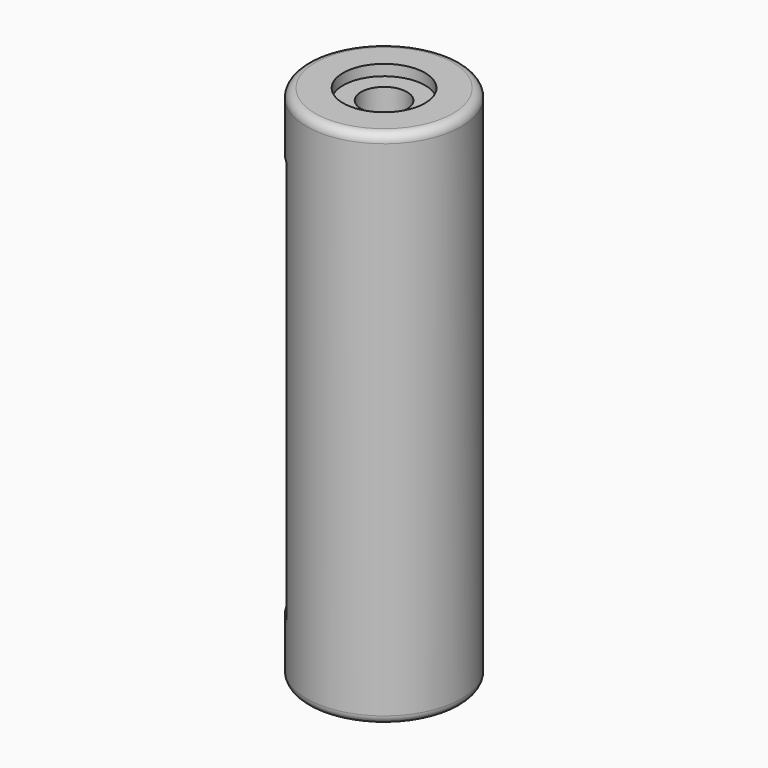
from build123d import *

# Parameters (mm, degrees)
F0_R          = 7.1
F0_R_2        = 2.1
F1_DEPTH      = 47.7
F3_DEPTH      = 3.2
F4_R          = 3.75
F5_DEPTH      = 1
F6_W          = 8
F6_H          = 35.7
F7_DEPTH      = 25
F9_START      = -2.5
F8_R          = 5.1
F9_DEPTH      = 37.5
F10_T1_DEPTH  = 35.7
F10_T8_ANGLE  = 100.8666218277
F10_T14_ANGLE = 100.8666218277
F10_T23_DEPTH = 40.4388611997
F10_T27_ANGLE = 100.8666218277
F10_T34_ANGLE = 100.8666218277
F10_T38_DEPTH = 40.4388611997
F10_T45_DEPTH = 40.4388611997
F10_T49_ANGLE = 100.8666218277
F10_T56_DEPTH = 40.4388611997
F10_T60_ANGLE = 100.8666218277


# Not quite as in the source:
# - a fillet or chamfer that OpenCascade refuses, or shapes differently, is made with other operations: its cross-section is extruded or revolved along the edge and cut away or added


with BuildPart() as f1:
    # F0 (on Top) → F1 (new body)
    with BuildSketch(Plane.XY):
        Circle(F0_R)
        Circle(F0_R_2, mode=Mode.SUBTRACT)
    extrude(amount=F1_DEPTH)

    # F2 (on face) → F3 (cut)
    with BuildSketch(Plane(origin=(0, 0, 0), x_dir=(1, 0, 0), z_dir=(0, 0, -1))):
        Polygon((2.6088002978, -3.8114950268), (4.6052516685, 0.3535398179), (1.9964513707, 4.1650348447), (-2.6088002978, 3.8114950268), (-4.6052516685, -0.3535398179), (-1.9964513707, -4.1650348447), align=None)
    extrude(amount=-F3_DEPTH, mode=Mode.SUBTRACT)

    # F4 (on face) → F5 (cut)
    with BuildSketch(Plane.XY.offset(47.7)):
        Circle(F4_R)
    extrude(amount=-F5_DEPTH, mode=Mode.SUBTRACT)

    # F6 (on Right) → F7 (cut)
    with BuildSketch(Plane.YZ):
        with Locations((0, 23.85)):
            Rectangle(F6_W, F6_H)
    extrude(amount=-F7_DEPTH, mode=Mode.SUBTRACT)

    # F8 (on face) → F9 (cut)
    with BuildSketch(Plane(origin=(0, 0, 3.2), x_dir=(1, 0, 0), z_dir=(0, 0, -1)).offset(F9_START)):
        Circle(F8_R)
    extrude(amount=-F9_DEPTH, mode=Mode.SUBTRACT)

    # F10: fillet of radius 0.8 on 6 edges, made by hand

    # F10_s2 → F10_t1 (cut)
    with BuildSketch(Plane.XY.offset(6)):
        with BuildLine():
            ThreePointArc((-4.5985924101, 5.4095238095), (-4.831313661, 4.5239737763), (-4.0804411526, 4))
            Line((-4.0804411526, 4), (-5.8660037504, 4))
            ThreePointArc((-5.8660037504, 4), (-5.279548517, 4.747248409), (-4.5985924101, 5.4095238095))
        make_face()
        with BuildLine():
            ThreePointArc((-4.5985924101, -5.4095238095), (-4.831313661, -4.5239737763), (-4.0804411526, -4))
            Line((-4.0804411526, -4), (-5.8660037504, -4))
            ThreePointArc((-5.8660037504, -4), (-5.279548517, -4.747248409), (-4.5985924101, -5.4095238095))
        make_face()
    extrude(amount=F10_T1_DEPTH, mode=Mode.SUBTRACT)

    # F10_s3 → F10_t4 (revolve, cut)
    with BuildSketch(Plane.XZ):
        with BuildLine():
            ThreePointArc((7.1, 0.8), (6.8656854249, 0.2343145751), (6.3, 0))
            Line((6.3, 0), (7.1, 0))
            Line((7.1, 0), (7.1, 0.8))
        make_face()
    revolve(axis=Axis((0, 0, 0), (0, 0, 1)), mode=Mode.SUBTRACT)


with BuildPart() as f10_tool6:
    # F10_s7 → F10_t8 (revolve)
    with BuildSketch(Plane(origin=(0, 0, 0), x_dir=(0, 0, 1), z_dir=(0.7708837014, -0.6369759171, 0))):
        with BuildLine():
            ThreePointArc((5.2, 7.1), (5.7656854249, 6.8656854249), (6, 6.3))
            Line((6, 6.3), (6, 7.1))
            Line((6, 7.1), (5.2, 7.1))
        make_face()
    revolve(axis=Axis((0, 0, 6), (0, 0, -1)), revolution_arc=F10_T8_ANGLE)

    split(bisect_by=Plane.XZ.offset(4), keep=Keep.BOTTOM)

    split(bisect_by=Plane.XZ.offset(-4), keep=Keep.TOP)


with BuildPart() as f1_1:
    add(f1.part)

    # F10_t5: cut F10_tool6
    add(f10_tool6.part, mode=Mode.SUBTRACT)


with BuildPart() as f10_tool12:
    # F10_s13 → F10_t14 (revolve)
    with BuildSketch(Plane(origin=(0, 0, 0), x_dir=(0, 0, 1), z_dir=(0.7708837014, -0.6369759171, 0))):
        with BuildLine():
            ThreePointArc((42.5, 7.1), (41.9343145751, 6.8656854249), (41.7, 6.3))
            Line((41.7, 6.3), (41.7, 7.1))
            Line((41.7, 7.1), (42.5, 7.1))
        make_face()
    revolve(axis=Axis((0, 0, 41.7), (0, 0, -1)), revolution_arc=F10_T14_ANGLE)

    split(bisect_by=Plane.XZ.offset(4), keep=Keep.BOTTOM)

    split(bisect_by=Plane.XZ.offset(-4), keep=Keep.TOP)


with BuildPart() as f1_2:
    add(f1_1.part)

    # F10_t11: cut F10_tool12
    add(f10_tool12.part, mode=Mode.SUBTRACT)

    # F10_s17 → F10_t18 (revolve, cut)
    with BuildSketch(Plane.XZ):
        with BuildLine():
            ThreePointArc((7.1, 46.9), (6.8656854249, 47.4656854249), (6.3, 47.7))
            Line((6.3, 47.7), (7.1, 47.7))
            Line((7.1, 47.7), (7.1, 46.9))
        make_face()
    revolve(axis=Axis((0, 0, 47.7), (0, 0, 1)), mode=Mode.SUBTRACT)


with BuildPart() as f10_tool21:
    # F10_s22 → F10_t23 (new body)
    with BuildSketch(Plane.XY.offset(41.7)):
        with BuildLine():
            ThreePointArc((-4.5985924101, -5.4095238095), (-4.831313661, -4.5239737763), (-4.0804411526, -4))
            Line((-4.0804411526, -4), (-5.8660037504, -4))
            ThreePointArc((-5.8660037504, -4), (-5.279548517, -4.747248409), (-4.5985924101, -5.4095238095))
        make_face()
    extrude(amount=-F10_T23_DEPTH)

    split(bisect_by=Plane.XY.offset(6), keep=Keep.BOTTOM)


with BuildPart() as f10_tool25:
    # F10_s26 → F10_t27 (revolve)
    with BuildSketch(Plane(origin=(0, 0, 0), x_dir=(0, 0, 1), z_dir=(0.7708837014, -0.6369759171, 0))):
        with BuildLine():
            ThreePointArc((5.2, 7.1), (5.7656854249, 6.8656854249), (6, 6.3))
            Line((6, 6.3), (6, 7.1))
            Line((6, 7.1), (5.2, 7.1))
        make_face()
    revolve(axis=Axis((0, 0, 6), (0, 0, -1)), revolution_arc=F10_T27_ANGLE)

    split(bisect_by=Plane.XZ.offset(4), keep=Keep.TOP)


with BuildPart() as f10_tool21_1:
    add(f10_tool21.part)

    # F10_t29: intersect F10_tool25
    add(f10_tool25.part, mode=Mode.INTERSECT)


with BuildPart() as f1_3:
    add(f1_2.part)

    # F10_t19: cut F10_tool21
    add(f10_tool21_1.part, mode=Mode.SUBTRACT)


with BuildPart() as f10_tool32:
    # F10_s33 → F10_t34 (revolve)
    with BuildSketch(Plane(origin=(0, 0, 0), x_dir=(0, 0, 1), z_dir=(0.7708837014, -0.6369759171, 0))):
        with BuildLine():
            ThreePointArc((5.2, 7.1), (5.7656854249, 6.8656854249), (6, 6.3))
            Line((6, 6.3), (6, 7.1))
            Line((6, 7.1), (5.2, 7.1))
        make_face()
    revolve(axis=Axis((0, 0, 6), (0, 0, -1)), revolution_arc=F10_T34_ANGLE)

    split(bisect_by=Plane.XZ.offset(-4), keep=Keep.BOTTOM)


with BuildPart() as f10_tool36:
    # F10_s37 → F10_t38 (new body)
    with BuildSketch(Plane.XY.offset(41.7)):
        with BuildLine():
            ThreePointArc((-4.5985924101, 5.4095238095), (-4.831313661, 4.5239737763), (-4.0804411526, 4))
            Line((-4.0804411526, 4), (-5.8660037504, 4))
            ThreePointArc((-5.8660037504, 4), (-5.279548517, 4.747248409), (-4.5985924101, 5.4095238095))
        make_face()
    extrude(amount=-F10_T38_DEPTH)

    split(bisect_by=Plane.XY.offset(6), keep=Keep.BOTTOM)


with BuildPart() as f10_tool32_1:
    add(f10_tool32.part)

    # F10_t40: intersect F10_tool36
    add(f10_tool36.part, mode=Mode.INTERSECT)


with BuildPart() as f1_4:
    add(f1_3.part)

    # F10_t30: cut F10_tool32
    add(f10_tool32_1.part, mode=Mode.SUBTRACT)


with BuildPart() as f10_tool43:
    # F10_s44 → F10_t45 (new body)
    with BuildSketch(Plane.XY.offset(46.4388611997)):
        with BuildLine():
            ThreePointArc((-4.5985924101, -5.4095238095), (-4.831313661, -4.5239737763), (-4.0804411526, -4))
            Line((-4.0804411526, -4), (-5.8660037504, -4))
            ThreePointArc((-5.8660037504, -4), (-5.279548517, -4.747248409), (-4.5985924101, -5.4095238095))
        make_face()
    extrude(amount=-F10_T45_DEPTH)

    split(bisect_by=Plane.XY.offset(41.7), keep=Keep.TOP)


with BuildPart() as f10_tool47:
    # F10_s48 → F10_t49 (revolve)
    with BuildSketch(Plane(origin=(0, 0, 0), x_dir=(0, 0, 1), z_dir=(0.7708837014, -0.6369759171, 0))):
        with BuildLine():
            ThreePointArc((42.5, 7.1), (41.9343145751, 6.8656854249), (41.7, 6.3))
            Line((41.7, 6.3), (41.7, 7.1))
            Line((41.7, 7.1), (42.5, 7.1))
        make_face()
    revolve(axis=Axis((0, 0, 41.7), (0, 0, -1)), revolution_arc=F10_T49_ANGLE)

    split(bisect_by=Plane.XZ.offset(4), keep=Keep.TOP)


with BuildPart() as f10_tool43_1:
    add(f10_tool43.part)

    # F10_t51: intersect F10_tool47
    add(f10_tool47.part, mode=Mode.INTERSECT)


with BuildPart() as f1_5:
    add(f1_4.part)

    # F10_t41: cut F10_tool43
    add(f10_tool43_1.part, mode=Mode.SUBTRACT)


with BuildPart() as f10_tool54:
    # F10_s55 → F10_t56 (new body)
    with BuildSketch(Plane.XY.offset(46.4388611997)):
        with BuildLine():
            ThreePointArc((-4.5985924101, 5.4095238095), (-4.831313661, 4.5239737763), (-4.0804411526, 4))
            Line((-4.0804411526, 4), (-5.8660037504, 4))
            ThreePointArc((-5.8660037504, 4), (-5.279548517, 4.747248409), (-4.5985924101, 5.4095238095))
        make_face()
    extrude(amount=-F10_T56_DEPTH)

    split(bisect_by=Plane.XY.offset(41.7), keep=Keep.TOP)


with BuildPart() as f10_tool58:
    # F10_s59 → F10_t60 (revolve)
    with BuildSketch(Plane(origin=(0, 0, 0), x_dir=(0, 0, 1), z_dir=(0.7708837014, -0.6369759171, 0))):
        with BuildLine():
            ThreePointArc((42.5, 7.1), (41.9343145751, 6.8656854249), (41.7, 6.3))
            Line((41.7, 6.3), (41.7, 7.1))
            Line((41.7, 7.1), (42.5, 7.1))
        make_face()
    revolve(axis=Axis((0, 0, 41.7), (0, 0, -1)), revolution_arc=F10_T60_ANGLE)

    split(bisect_by=Plane.XZ.offset(-4), keep=Keep.BOTTOM)


with BuildPart() as f10_tool54_1:
    add(f10_tool54.part)

    # F10_t62: intersect F10_tool58
    add(f10_tool58.part, mode=Mode.INTERSECT)


with BuildPart() as f1_6:
    add(f1_5.part)

    # F10_t52: cut F10_tool54
    add(f10_tool54_1.part, mode=Mode.SUBTRACT)


solid = f1_6.part
